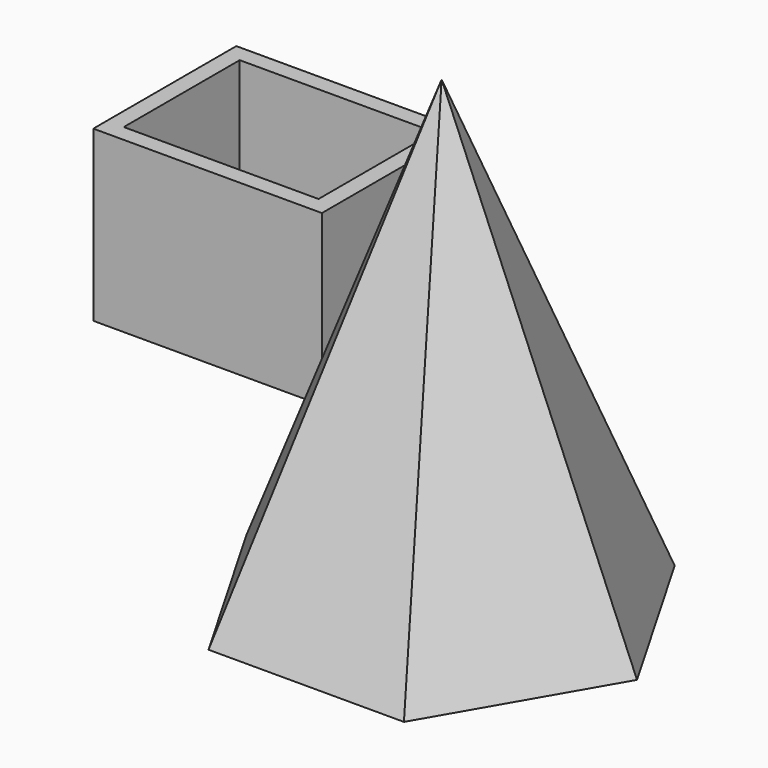
from build123d import *

# Parameters (mm, degrees)
F0_W     = 50.8
F0_H     = 50.8
F1_DEPTH = 53.975
F5_R     = 11.43
F6_DEPTH = 25.4
F7_W     = 34.3122780323
F7_H     = 26.8259719014
F8_DEPTH = 25.4
F9_T     = -2.54


# Not quite as in the source:
# - an extrude whose draft closes it to a point is written as a loft to that point


with BuildPart() as f1:
    # F0 (on Front) → F1 (new body, symmetric)
    with BuildSketch(Plane.XZ):
        with Locations((-25.4, 25.4)):
            Rectangle(F0_W, F0_H)
    extrude(amount=F1_DEPTH, both=True)


with BuildPart() as f4:
    # F3 (on Top) → F4 section 0
    with BuildSketch(Plane.XY, mode=Mode.PRIVATE) as f4_s0:
        Polygon((14.6646968374, 25.4), (-14.6646968374, 25.4), (-29.3293936748, 0), (-14.6646968374, -25.4), (14.6646968374, -25.4), (29.3293936748, 0), align=None)
    loft([f4_s0.sketch, Vertex(0, 0, 69.7859264541)], ruled=True)

    # F5 (on face) → F6 (cut)
    with BuildSketch(Plane(origin=(0, 0, 0), x_dir=(1, 0, 0), z_dir=(0, 0, -1))):
        Circle(F5_R)
    extrude(amount=-F6_DEPTH, mode=Mode.SUBTRACT)


with BuildPart() as f8:
    # F7 (on Top) → F8 (new body)
    with BuildSketch(Plane.XY):
        with Locations((-60.2024570107, 44.761929661)):
            Rectangle(F7_W, F7_H)
    extrude(amount=F8_DEPTH)

    # F9
    f9_openings = [f8.faces().sort_by_distance(p)[0] for p in [
        (-60.202457, 44.76193, 25.4),
    ]]
    offset(amount=F9_T, openings=f9_openings)


solid = Compound([f4.part, f8.part])
